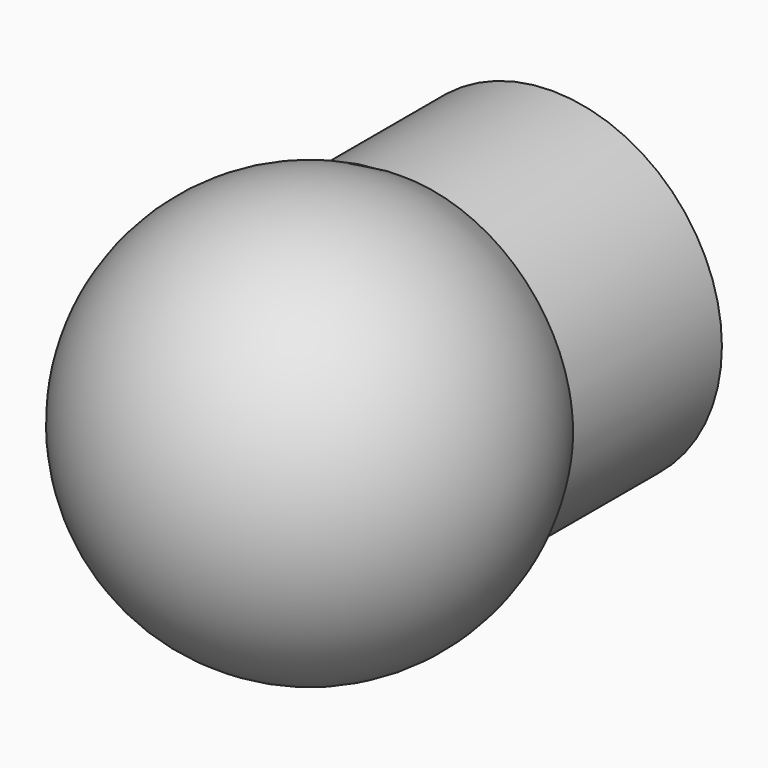
from build123d import *

# Parameters (mm, degrees)
F0_R     = 14
F0_R_2   = 11.6
F1_DEPTH = 25
F2_D     = 12.7
F2_DEPTH = 14
F2_TIP   = 3.8154649308


# Not quite as in the source:
# - a length typed as a fraction of an inch, garbled in the dataset ("3 / 203.2 mm" for 3/8 in), is restored


with BuildPart() as f1:
    # F0 (on Front) → F1 (new body)
    with BuildSketch(Plane.XZ):
        Circle(F0_R)
        Circle(F0_R_2, mode=Mode.SUBTRACT)
        Circle(F0_R_2)
    extrude(amount=F1_DEPTH)

    # F2
    with Locations(Plane(origin=(0, 0, 0), x_dir=(1, 0, 0), z_dir=(0, 1, 0))):
        with Locations((0, 0)):
            Hole(F2_D / 2, depth=F2_DEPTH)
            with Locations((0, 0, -(F2_DEPTH + F2_TIP / 2))):  # 118° drill point
                Cone(0, F2_D / 2, F2_TIP, mode=Mode.SUBTRACT)

    # F3 (on face) → F4 (revolve)
    with BuildSketch(Plane.XZ.offset(25)):
        with BuildLine():
            Line((17, 0), (14, 0))
            ThreePointArc((14, 0), (0, -14), (-14, 0))
            Line((-14, 0), (-17, 0))
            ThreePointArc((-17, 0), (0, -17), (17, 0))
        make_face()
        with BuildLine():
            ThreePointArc((-14, 0), (0, -14), (14, 0))
            Line((14, 0), (-14, 0))
        make_face()
    revolve(axis=Axis((0, -25, 0), (1, 0, 0)))


solid = f1.part
